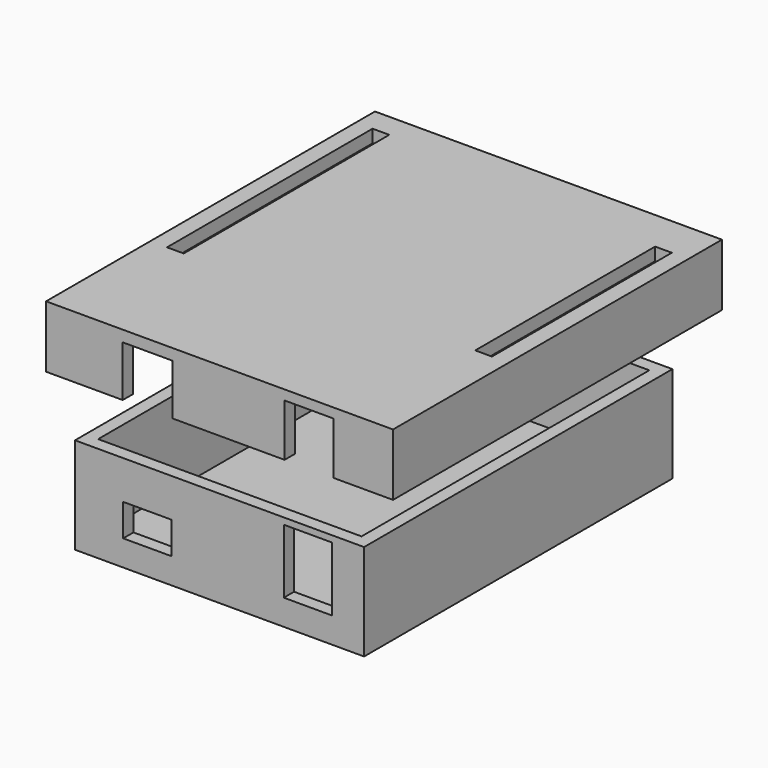
from build123d import *

# Parameters (mm, degrees)
F0_W      = 57.15
F0_H      = 19.05
F1_DEPTH  = 76.2
F2_T      = -2.54
F3_W      = 9.525
F3_H      = 6.35
F4_DEPTH  = 25.4
F5_W      = 9.525
F5_H      = 12.7
F6_DEPTH  = 25.4
F8_W      = 68.5918703675
F8_H      = 12.2578628361
F9_DEPTH  = 81.28
F10_T     = -2.54
F11_W     = 9.833057411
F11_H     = 10.0466273725
F11_W_2   = 9.6692787483
F11_H_2   = 10.3357378393
F12_DEPTH = 25.4
F13_W     = 3.302
F13_H     = 50.8
F14_DEPTH = 25.4
F15_W     = 3.302
F15_H     = 44.45
F16_DEPTH = 25.4


with BuildPart() as f1:
    # F0 (on Front) → F1 (new body)
    with BuildSketch(Plane.XZ):
        Rectangle(F0_W, F0_H)
    extrude(amount=F1_DEPTH)

    # F2
    f2_openings = [f1.faces().sort_by_distance(p)[0] for p in [
        (0, -38.1, 9.525),
    ]]
    offset(amount=F2_T, openings=f2_openings)

    # F3 (on face) → F4 (cut)
    with BuildSketch(Plane.XZ.offset(76.2)):
        with Locations((-14.2875, -1.27)):
            Rectangle(F3_W, F3_H)
    extrude(amount=-F4_DEPTH, mode=Mode.SUBTRACT)

    # F5 (on face) → F6 (cut)
    with BuildSketch(Plane.XZ.offset(76.2)):
        with Locations((17.4625, 1.905)):
            Rectangle(F5_W, F5_H)
    extrude(amount=-F6_DEPTH, mode=Mode.SUBTRACT)


with BuildPart() as f9:
    # F8 (on face) → F9 (new body)
    with BuildSketch(Plane.XZ.offset(76.2)):
        with Locations((0, 25.7245693356)):
            Rectangle(F8_W, F8_H)
    extrude(amount=-F9_DEPTH)

    # F10
    f10_openings = [f9.faces().sort_by_distance(p)[0] for p in [
        (0, -35.56, 19.595638),
    ]]
    offset(amount=F10_T, openings=f10_openings)

    # F11 (on face) → F12 (cut)
    with BuildSketch(Plane.XZ.offset(76.2)):
        with Locations((-14.2288259231, 24.6189516038)):
            Rectangle(F11_W, F11_H)
        with Locations((17.6961715333, 24.7635068372)):
            Rectangle(F11_W_2, F11_H_2)
    extrude(amount=-F12_DEPTH, mode=Mode.SUBTRACT)

    # F13 (on face) → F14 (cut)
    with BuildSketch(Plane.XY.offset(31.8535007536)):
        with Locations((-29.3429351838, -25.0374122988)):
            Rectangle(F13_W, F13_H)
    extrude(amount=-F14_DEPTH, mode=Mode.SUBTRACT)

    # F15 (on face) → F16 (cut)
    with BuildSketch(Plane.XY.offset(31.8535007536)):
        with Locations((29.3429351838, -25.4)):
            Rectangle(F15_W, F15_H)
    extrude(amount=-F16_DEPTH, mode=Mode.SUBTRACT)


solid = Compound([f1.part, f9.part])
